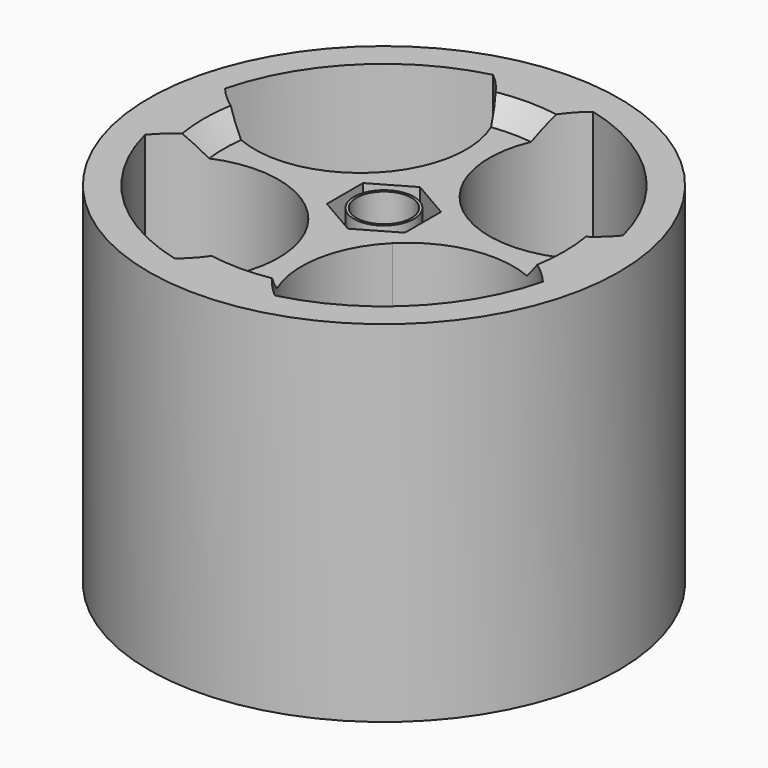
from build123d import *

# Parameters (mm, degrees)
F0_R     = 23.5
F0_R_2   = 22.5
F0_R_3   = 3
F1_DEPTH = 35
F2_START = 2
F0_R_4   = 2.75
F2_DEPTH = 31
F4_DEPTH = 6
F5_START = 23
F5_DEPTH = 12


# Not quite as in the source:
# - a fillet or chamfer that OpenCascade refuses, or shapes differently, is made with other operations: its cross-section is extruded or revolved along the edge and cut away or added


with BuildPart() as f1:
    # F0 (on Top) → F1 (new body)
    with BuildSketch(Plane.XY):
        Circle(F0_R)
        Circle(F0_R_2, mode=Mode.SUBTRACT)
        Circle(F0_R_2)
        with BuildLine():
            ThreePointArc((19.8808953521, 5), (20.3446351002, 2.5190916302), (20.5, 0))
            ThreePointArc((20.5, 0), (20.3446351002, -2.5190916302), (19.8808953521, -5))
            ThreePointArc((19.8808953521, -5), (14.4956890143, -14.4956890143), (5, -19.8808953521))
            ThreePointArc((5, -19.8808953521), (0, -20.5), (-5, -19.8808953521))
            ThreePointArc((-5, -19.8808953521), (-14.4956890143, -14.4956890143), (-19.8808953521, -5))
            ThreePointArc((-19.8808953521, -5), (-20.5, 0), (-19.8808953521, 5))
            ThreePointArc((-19.8808953521, 5), (-14.4956890143, 14.4956890143), (-5, 19.8808953521))
            ThreePointArc((-5, 19.8808953521), (0, 20.5), (5, 19.8808953521))
            ThreePointArc((5, 19.8808953521), (14.4956890143, 14.4956890143), (19.8808953521, 5))
        make_face(mode=Mode.SUBTRACT)
        with BuildLine():
            ThreePointArc((6, 0), (5.5432771953, 2.2961005937), (4.2426406878, 4.2426406864))
            ThreePointArc((4.2426406878, 4.2426406864), (7.8e-09, 6), (-4.2426406768, 4.2426406974))
            ThreePointArc((-4.2426406768, 4.2426406974), (-6, 7.9e-09), (-4.242640688, -4.2426406862))
            ThreePointArc((-4.242640688, -4.2426406862), (-1.21e-08, -6), (4.2426406709, -4.2426407033))
            ThreePointArc((4.2426406709, -4.2426407033), (5.5432771907, -2.2961006048), (6, 0))
        make_face()
        Polygon((-3.9, -2.2516660498), (-3.9, 2.2516660498), (0, 4.5033320997), (3.9, 2.2516660498), (3.9, -2.2516660498), (0, -4.5033320997), align=None, mode=Mode.SUBTRACT)
        with BuildLine():
            ThreePointArc((4.2426406878, 4.2426406864), (1.1585914251, 12.2294676794), (5, 19.8808953521))
            ThreePointArc((5, 19.8808953521), (0, 20.5), (-5, 19.8808953521))
            ThreePointArc((-5, 19.8808953521), (-1.1585914255, 12.2294676871), (-4.2426406768, 4.2426406974))
            ThreePointArc((-4.2426406768, 4.2426406974), (7.8e-09, 6), (4.2426406878, 4.2426406864))
        make_face()
        with BuildLine():
            ThreePointArc((19.8808953521, -5), (20.3446351002, -2.5190916302), (20.5, 0))
            ThreePointArc((20.5, 0), (20.3446351002, 2.5190916302), (19.8808953521, 5))
            ThreePointArc((19.8808953521, 5), (12.2294676803, 1.1585914252), (4.2426406878, 4.2426406864))
            ThreePointArc((4.2426406878, 4.2426406864), (5.5432771953, 2.2961005937), (6, 0))
            ThreePointArc((6, 0), (5.5432771907, -2.2961006048), (4.2426406709, -4.2426407033))
            ThreePointArc((4.2426406709, -4.2426407033), (12.2294676684, -1.1585914246), (19.8808953521, -5))
        make_face()
        with BuildLine():
            ThreePointArc((-5, -19.8808953521), (0, -20.5), (5, -19.8808953521))
            ThreePointArc((5, -19.8808953521), (1.1585914257, -12.2294676913), (4.2426406709, -4.2426407033))
            ThreePointArc((4.2426406709, -4.2426407033), (-1.21e-08, -6), (-4.242640688, -4.2426406862))
            ThreePointArc((-4.242640688, -4.2426406862), (-1.1585914251, -12.2294676792), (-5, -19.8808953521))
        make_face()
        with BuildLine():
            ThreePointArc((-4.242640688, -4.2426406862), (-6, 7.9e-09), (-4.2426406768, 4.2426406974))
            ThreePointArc((-4.2426406768, 4.2426406974), (-12.2294676726, 1.1585914248), (-19.8808953521, 5))
            ThreePointArc((-19.8808953521, 5), (-20.5, 0), (-19.8808953521, -5))
            ThreePointArc((-19.8808953521, -5), (-12.2294676805, -1.1585914252), (-4.242640688, -4.2426406862))
        make_face()
        Polygon((0, 4.5033320997), (-3.9, 2.2516660498), (-3.9, -2.2516660498), (0, -4.5033320997), (3.9, -2.2516660498), (3.9, 2.2516660498), align=None)
        Circle(F0_R_3, mode=Mode.SUBTRACT)
    extrude(amount=F1_DEPTH)

    # F0 (on Top) → F2 (join)
    with BuildSketch(Plane.XY.offset(F2_START)):
        Circle(F0_R_3)
        Circle(F0_R_4, mode=Mode.SUBTRACT)
    extrude(amount=F2_DEPTH)

    # F3: chamfer of 15 on 1 edges, made by hand


with BuildPart() as f3_tool2:
    # F3_s3 → F3_t4 (revolve)
    with BuildSketch(Plane.XZ):
        Polygon((18, 35), (3, 20), (3, 35), align=None)
    revolve(axis=Axis((0, 0, 35), (0, 0, 1)))

    split(bisect_by=Plane.XY.offset(33), keep=Keep.TOP)


with BuildPart() as f1_1:
    add(f1.part)

    # F3_t1: cut F3_tool2
    add(f3_tool2.part, mode=Mode.SUBTRACT)

    # F0 (on Top) → F4 (cut)
    with BuildSketch(Plane.XY):
        Polygon((0, 4.5033320997), (-3.9, 2.2516660498), (-3.9, -2.2516660498), (0, -4.5033320997), (3.9, -2.2516660498), (3.9, 2.2516660498), align=None)
        Circle(F0_R_3, mode=Mode.SUBTRACT)
    extrude(amount=F4_DEPTH, mode=Mode.SUBTRACT)

    # F0 (on Top) → F5 (cut)
    with BuildSketch(Plane.XY.offset(F5_START)):
        Polygon((0, 4.5033320997), (-3.9, 2.2516660498), (-3.9, -2.2516660498), (0, -4.5033320997), (3.9, -2.2516660498), (3.9, 2.2516660498), align=None)
        Circle(F0_R_3, mode=Mode.SUBTRACT)
    extrude(amount=F5_DEPTH, mode=Mode.SUBTRACT)


solid = f1_1.part
